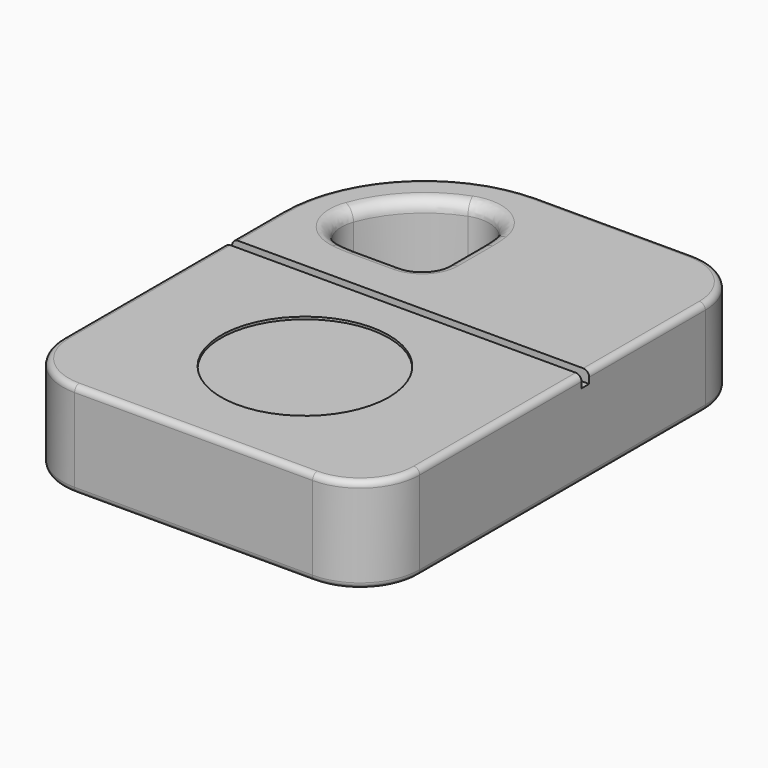
from build123d import *

# Parameters (mm, degrees)
F0_W        = 30
F0_H        = 40
F1_DEPTH    = 8
F2_R        = 12
F3_R        = 5
F5_DEPTH    = 25
F4_W        = 26.9999996879
F4_H        = 0.8
F4_W_2      = 3.0000003121
F6_DEPTH    = 1
F7_T1_DEPTH = 8
F8_R        = 3
F9_R        = 2
F10_R       = 0.5
F11_R       = 1
F12_R       = 7.0500114294
F13_DEPTH   = 0.2


# Not quite as in the source:
# - a fillet or chamfer that OpenCascade refuses, or shapes differently, is made with other operations: its cross-section is extruded or revolved along the edge and cut away or added


with BuildPart() as f1:
    # F0 (on Top) → F1 (new body)
    with BuildSketch(Plane.XY):
        with Locations((15, -20)):
            Rectangle(F0_W, F0_H)
    extrude(amount=F1_DEPTH)

    # F2
    f2_edges = [f1.edges().sort_by_distance(p)[0] for p in [
        (0, 0, 4),
    ]]
    fillet(f2_edges, radius=F2_R)

    # F3
    f3_edges = [f1.edges().sort_by_distance(p)[0] for p in [
        (30, 0, 4),
        (30, -40, 4),
        (0, -40, 4),
    ]]
    fillet(f3_edges, radius=F3_R)

    # F4 (on face) → F5 (cut)
    with BuildSketch(Plane.XY.offset(8)):
        with BuildLine():
            Line((3.0000003121, -12), (3.0000003121, -13.0000003121))
            Line((3.0000003121, -13.0000003121), (13.0000003121, -13.0000003121))
            Line((13.0000003121, -13.0000003121), (13.0000003121, -3.0000003121))
            Line((13.0000003121, -3.0000003121), (12, -3.0000003121))
            ThreePointArc((12, -3.0000003121), (5.63603919, -5.63603919), (3.0000003121, -12))
        make_face()
    extrude(amount=-F5_DEPTH, mode=Mode.SUBTRACT)

    # F4 (on face) → F6 (cut)
    with BuildSketch(Plane.XY.offset(8)):
        with Locations((16.500000156, -17.6)):
            Rectangle(F4_W, F4_H)
        with Locations((1.500000156, -17.6)):
            Rectangle(F4_W_2, F4_H)
    extrude(amount=-F6_DEPTH, mode=Mode.SUBTRACT)

    # F7: fillet of radius 10 on 2 edges, made by hand

    # F7_s2 → F7_t1 (join)
    with BuildSketch(Plane.XY):
        with BuildLine():
            ThreePointArc((13.0000003121, -7.3588999), (12.7467945768, -5.1228315736), (12, -3.0000003121))
            Line((12, -3.0000003121), (13.0000003121, -3.0000003121))
            Line((13.0000003121, -3.0000003121), (13.0000003121, -7.3588999))
        make_face()
        with BuildLine():
            ThreePointArc((3.0000003121, -12), (5.1228315736, -12.7467945768), (7.3588999, -13.0000003121))
            Line((7.3588999, -13.0000003121), (3.0000003121, -13.0000003121))
            Line((3.0000003121, -13.0000003121), (3.0000003121, -12))
        make_face()
    extrude(amount=F7_T1_DEPTH)

    # F8
    f8_edges = [f1.edges().sort_by_distance(p)[0] for p in [
        (12, -3, 4),
        (3, -12, 4),
    ]]
    fillet(f8_edges, radius=F8_R)

    # F9
    f9_edges = [f1.edges().sort_by_distance(p)[0] for p in [
        (13, -13, 4),
    ]]
    fillet(f9_edges, radius=F9_R)

    # F10
    f10_edges = [f1.edges().sort_by_distance(p)[0] for p in [
        (30, -11.1, 8),
        (30, -26.5, 8),
        (30, -20, 0),
        (18.5, 0, 0),
        (3.514719, -3.514719, 0),
        (0, -23.5, 0),
        (1.464466, -38.535534, 0),
        (15, -40, 0),
        (28.535534, -38.535534, 0),
        (28.535534, -1.464466, 0),
        (18.5, 0, 8),
        (3.514719, -3.514719, 8),
        (0, -26.5, 8),
        (0, -14.6, 8),
        (1.464466, -38.535534, 8),
        (15, -40, 8),
        (28.535534, -38.535534, 8),
        (28.535534, -1.464466, 8),
    ]]
    fillet(f10_edges, radius=F10_R)

    # F11
    f11_edges = [f1.edges().sort_by_distance(p)[0] for p in [
        (5.636039, -5.636039, 8),
        (11.467525, -3.792736, 0),
        (9.17945, -13, 0),
        (12.414214, -12.414214, 0),
        (6.649711, -12.974821, 0),
        (13, -9.17945, 0),
        (3.792736, -11.467525, 0),
        (12.974821, -6.649711, 0),
        (5.636039, -5.636039, 0),
        (9.17945, -13, 8),
        (12.414214, -12.414214, 8),
        (6.649711, -12.974821, 8),
        (13, -9.17945, 8),
        (3.792736, -11.467525, 8),
        (12.974821, -6.649711, 8),
        (11.467525, -3.792736, 8),
    ]]
    fillet(f11_edges, radius=F11_R)

    # F12 (on face) → F13 (cut)
    with BuildSketch(Plane.XY.offset(8)):
        with Locations((15.0601761416, -28.3769778907)):
            Circle(F12_R)
    extrude(amount=-F13_DEPTH, mode=Mode.SUBTRACT)


solid = f1.part
